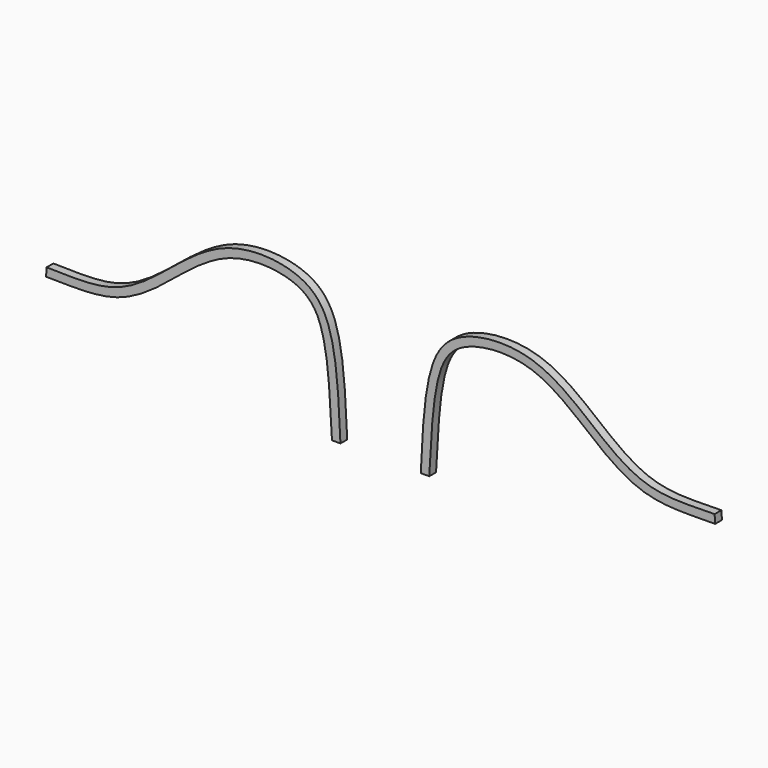
from build123d import *

# Parameters (mm, degrees)
F1_DEPTH = 1.5875


# Not quite as in the source:
# - a length typed as a fraction of an inch, garbled in the dataset ("3 / 203.2 mm" for 3/8 in), is restored


with BuildPart() as f1:
    # F0 (on Front) → F1 (new body)
    with BuildSketch(Plane.XZ):
        with BuildLine():
            Line((-9.1143716127, 0), (-7.5268716127, 0))
            add(Edge.make_bspline(
                [(-7.5268716127, 0), (-7.8897503094, 7.7291327478), (-8.3889565818, 20.2458286021), (-15.9660956947, 26.4335907496), (-29.9202055315, 27.0183201289), (-41.1758854937, 16.7482591558), (-50.4303761466, 10.5875251753), (-58.4748027147, 11.1036899728), (-62.5999122858, 11.1537828535)],
                knots=[0, 0, 0, 0, 0.2084827091, 0.3420372599, 0.5075321761, 0.6875133158, 0.8401089973, 1, 1, 1, 1], degree=3))
            Line((-62.5999122858, 11.1537828535), (-62.6944303513, 9.5662828535))
            add(Edge.make_bspline(
                [(-9.1143716127, 0), (-9.5316806414, 7.4013263291), (-9.9538721904, 19.2809836646), (-16.2634207351, 24.7436120288), (-29.273146146, 25.528857291), (-40.1716605131, 15.515392704), (-49.838939503, 9.0301520056), (-58.4163464612, 9.5533290209), (-62.6944303513, 9.5662828535)],
                knots=[0, 0, 0, 0, 0.2071362327, 0.3321209014, 0.4936369942, 0.6739603513, 0.8330255453, 1, 1, 1, 1], degree=3))
        make_face()
    extrude(amount=F1_DEPTH)


with BuildPart() as f1b:
    # F0 (on Front) → F1, piece 2 (new body)
    with BuildSketch(Plane.XZ):
        with BuildLine():
            add(Edge.make_bspline(
                [(7.5268716127, 0), (7.8897503094, 7.7291327478), (8.3889565818, 20.2458286021), (15.9660956947, 26.4335907496), (29.9202055315, 27.0183201289), (41.1758854937, 16.7482591558), (50.4303761466, 10.5875251753), (58.4748027147, 11.1036899728), (62.5999122858, 11.1537828535)],
                knots=[0, 0, 0, 0, 0.2084827091, 0.3420372599, 0.5075321761, 0.6875133158, 0.8401089973, 1, 1, 1, 1], degree=3))
            Line((7.5268716127, 0), (9.1143716127, 0))
            add(Edge.make_bspline(
                [(9.1143716127, 0), (9.5316806414, 7.4013263291), (9.9538721904, 19.2809836646), (16.2634207351, 24.7436120288), (29.273146146, 25.528857291), (40.1716605131, 15.515392704), (49.838939503, 9.0301520056), (58.4163464612, 9.5533290209), (62.6944303513, 9.5662828535)],
                knots=[0, 0, 0, 0, 0.2071362327, 0.3321209014, 0.4936369942, 0.6739603513, 0.8330255453, 1, 1, 1, 1], degree=3))
            Line((62.6944303513, 9.5662828535), (62.5999122858, 11.1537828535))
        make_face()
    extrude(amount=F1_DEPTH)


solid = Compound([f1.part, f1b.part])
